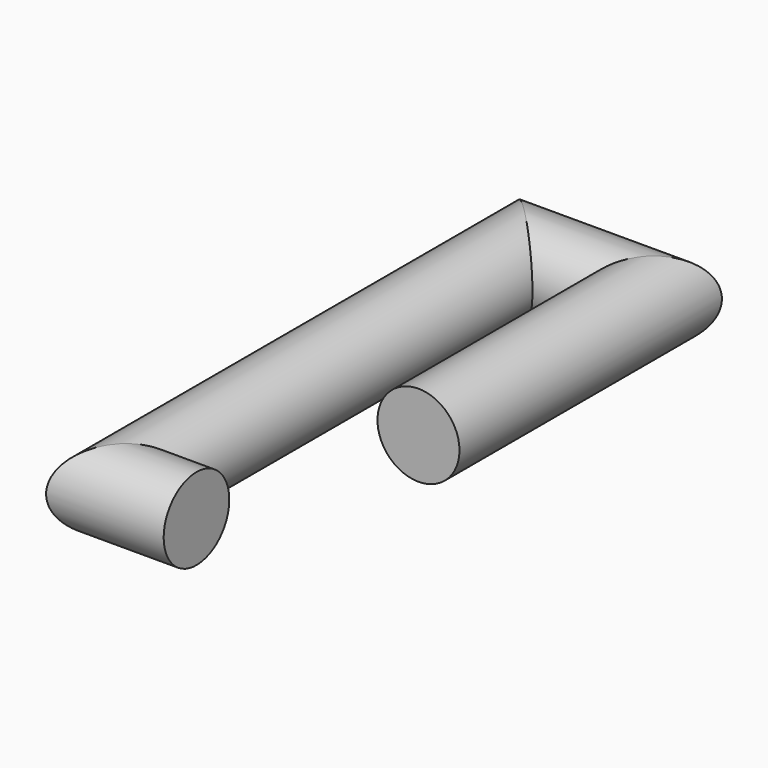
from build123d import *

# Parameters (mm, degrees)
F0_R = 5


with BuildPart() as f2:
    # F2: sweep along a path in F1
    with BuildLine(Plane.XY) as f2_path:
        Line((0, 0), (0, 35.0061804056))
        Line((0, 35.0061804056), (-15.1096209884, 35.0061804056))
        Line((-15.1096209884, 35.0061804056), (-15.1096209884, -26.629941538))
        Line((-15.1096209884, -26.629941538), (-5.7708141394, -26.629941538))
    # F0 (on Front) → F2 (sweep)
    with BuildSketch(Plane.XZ):
        Circle(F0_R)
    sweep(path=f2_path.line, transition=Transition.RIGHT)


solid = f2.part
